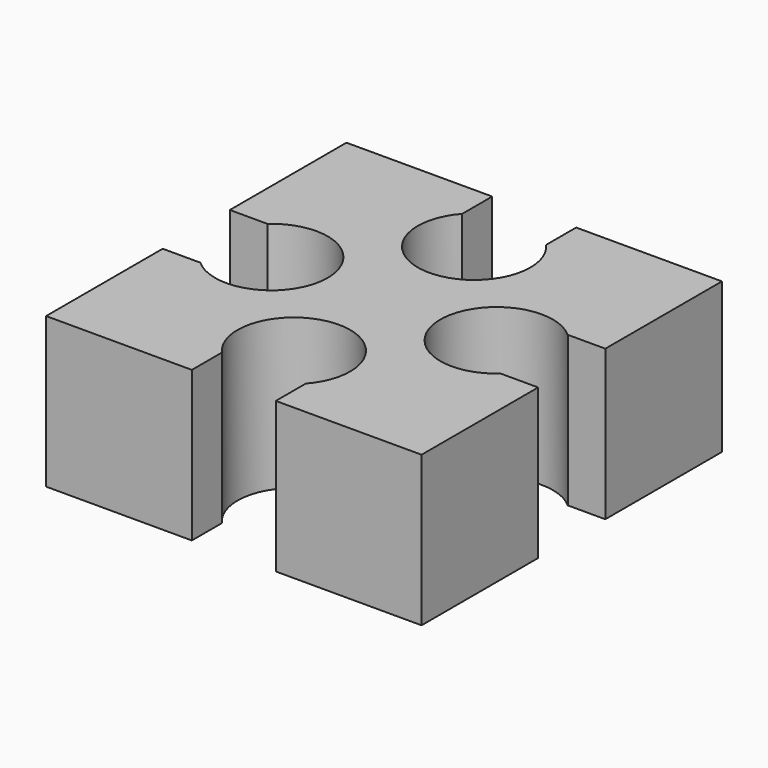
from build123d import *

# Parameters (mm, degrees)
F0_W            = 25.4
F0_H            = 25.4
F1_DEPTH        = 10.16
F2_R            = 3.81
F3_DEPTH        = 25.4
F3_COPIES_COUNT = 4
F5_DEPTH        = 25.4
F5_COPIES_COUNT = 4


# Not quite as in the source:
# - a pattern or mirror of a feature is missing from the dataset's text; its kind, count and spacing are read off the source's solid


with BuildPart() as f1:
    # F0 (on Top) → F1 (new body)
    with BuildSketch(Plane.XY):
        Rectangle(F0_W, F0_H)
    extrude(amount=F1_DEPTH)

    # F2 (on face) → F3 (cut)
    with BuildSketch(Plane.XY.offset(10.16)):
        with Locations((0, -7.62)):
            Circle(F2_R)
    f3 = extrude(amount=-F3_DEPTH, mode=Mode.SUBTRACT)

    # F3_copies: F3 ×4 about axis
    f3_copies_axis = Axis((0, 0, 0), (0, 0, 1))
    for i in range(1, F3_COPIES_COUNT):
        add(f3.rotate(f3_copies_axis, i * 360 / F3_COPIES_COUNT), mode=Mode.SUBTRACT)

    # F4 (on face) → F5 (cut)
    with BuildSketch(Plane.XY.offset(10.16)):
        with BuildLine():
            Line((-2.8398063314, -10.16), (-2.8398063314, -12.7))
            Line((-2.8398063314, -12.7), (2.8398063314, -12.7))
            Line((2.8398063314, -12.7), (2.8398063314, -10.16))
            ThreePointArc((2.8398063314, -10.16), (0, -11.43), (-2.8398063314, -10.16))
        make_face()
    f5 = extrude(amount=-F5_DEPTH, mode=Mode.SUBTRACT)

    # F5_copies: F5 ×4 about axis
    f5_copies_axis = Axis((0, 0, 0), (0, 0, 1))
    for i in range(1, F5_COPIES_COUNT):
        add(f5.rotate(f5_copies_axis, i * 360 / F5_COPIES_COUNT), mode=Mode.SUBTRACT)


solid = f1.part
